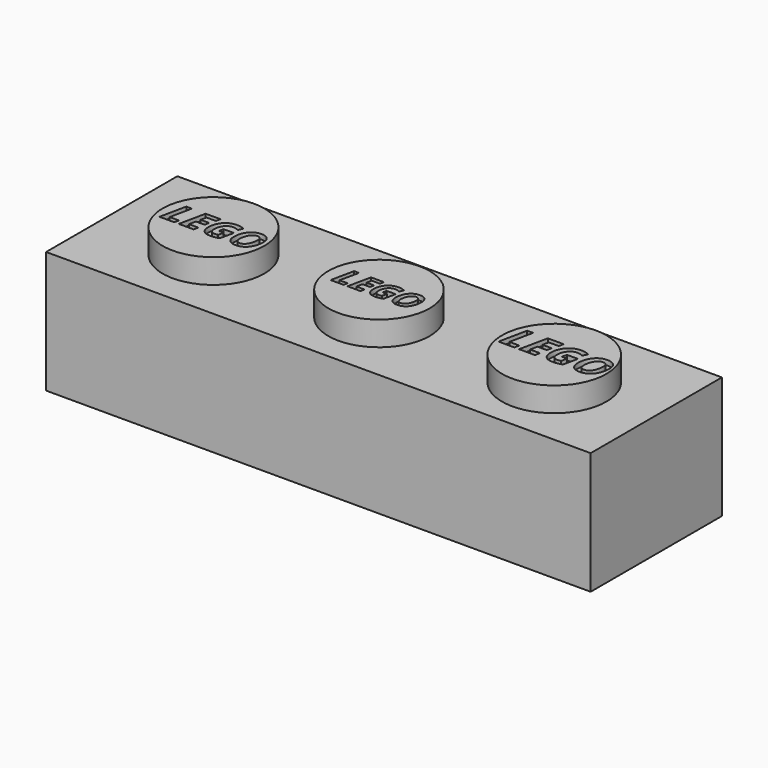
from build123d import *

# Parameters (mm, degrees)
F0_W          = 111.5427911282
F0_H          = 33.6096119136
F1_DEPTH      = 25
F2_R          = 10.4051525407
F3_DEPTH      = 5
F4_TEXT_SIZE  = 7.6294702012
F5_DEPTH      = 1
F6_W          = 101.1433741078
F6_H          = 23.4835067531
F7_DEPTH      = 23.2
F8_R          = 10.374305913
F8_R_2        = 10.696374041
F9_DEPTH      = 5
F10_TEXT_SIZE = 6.6705209772
F11_DEPTH     = 1
F12_TEXT_SIZE = 8.1500624755
F13_DEPTH     = 1
F14_R         = 3.0606556003
F15_DEPTH     = 1


# Not quite as in the source:
# - Text() gives the source's letters only with a copy of the font that has no kerning and outlines rounded to 1/6400 em; it was checked with that copy


with BuildPart() as f1:
    # F0 (on Top) → F1 (new body)
    with BuildSketch(Plane.XY):
        with Locations((-42.9219380021, 9.639990516)):
            Rectangle(F0_W, F0_H)
    extrude(amount=F1_DEPTH)

    # F2 (on face) → F3 (join)
    with BuildSketch(Plane.XY.offset(25)):
        with Locations((-77.1606490016, 8.7707350031)):
            Circle(F2_R)
    extrude(amount=F3_DEPTH)

    # F4 (on face) → F5 (cut)
    with BuildSketch(Plane.XY.offset(30)):
        with Locations((-86.352357514, 6.1858042299)):
            Text('LEGO', F4_TEXT_SIZE, font='Open Sans', font_style=FontStyle.BOLDITALIC, text_align=(TextAlign.LEFT, TextAlign.BOTTOM))
    extrude(amount=-F5_DEPTH, mode=Mode.SUBTRACT)

    # F6 (on face) → F7 (cut)
    with BuildSketch(Plane(origin=(0, 0, 0), x_dir=(1, 0, 0), z_dir=(0, 0, -1))):
        with Locations((-43.1973789819, -10.2783891489)):
            Rectangle(F6_W, F6_H)
    extrude(amount=-F7_DEPTH, mode=Mode.SUBTRACT)

    # F8 (on face) → F9 (join)
    with BuildSketch(Plane.XY.offset(25)):
        with Locations((-42.9669730365, 8.4118386731)):
            Circle(F8_R)
        with Locations((-7.0237480104, 8.3551155403)):
            Circle(F8_R_2)
    extrude(amount=F9_DEPTH)

    # F10 (on face) → F11 (cut)
    with BuildSketch(Plane.XY.offset(30)):
        with Locations((-51.2613095343, 6.1739212833)):
            Text('LEGO', F10_TEXT_SIZE, font='Open Sans', font_style=FontStyle.BOLDITALIC, text_align=(TextAlign.LEFT, TextAlign.BOTTOM))
    extrude(amount=-F11_DEPTH, mode=Mode.SUBTRACT)

    # F12 (on face) → F13 (cut)
    with BuildSketch(Plane.XY.offset(30)):
        with Locations((-17.0179624833, 6.2986443398)):
            Text('LEGO', F12_TEXT_SIZE, font='Open Sans', font_style=FontStyle.BOLDITALIC, text_align=(TextAlign.LEFT, TextAlign.BOTTOM))
    extrude(amount=-F13_DEPTH, mode=Mode.SUBTRACT)

    # F14 (on face) → F15 (cut)
    with BuildSketch(Plane(origin=(0, 0, 23.2), x_dir=(1, 0, 0), z_dir=(0, 0, -1))):
        with Locations((-43.1973785162, -9.7037917003)):
            Circle(F14_R)
    extrude(amount=-F15_DEPTH, mode=Mode.SUBTRACT)


solid = f1.part
